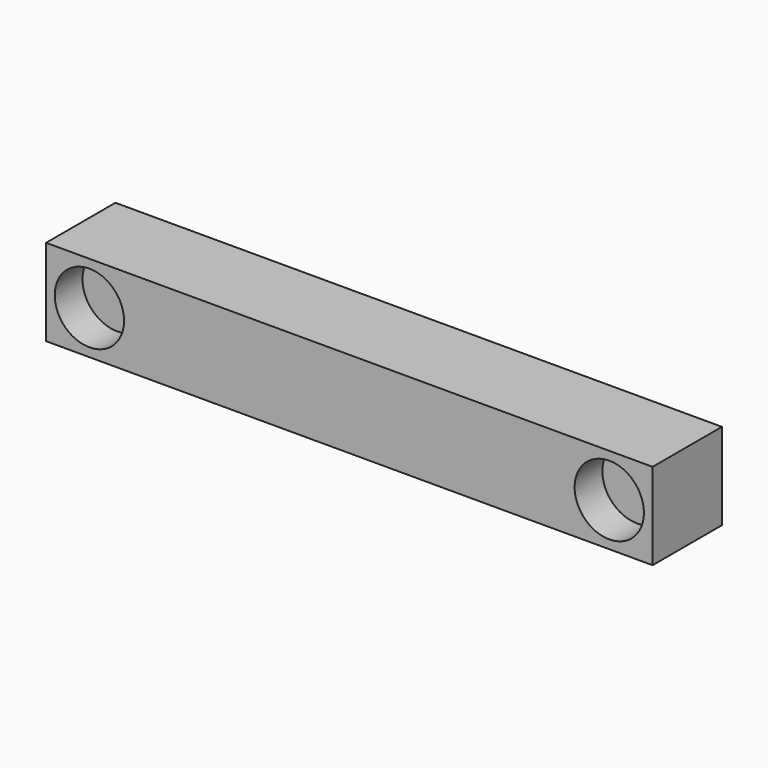
from build123d import *

# Parameters (mm, degrees)
F0_W     = 70
F0_H     = 10
F1_DEPTH = 10
F2_R     = 4
F3_DEPTH = 4


with BuildPart() as f1:
    # F0 (on Top) → F1 (new body)
    with BuildSketch(Plane.XY):
        with Locations((0, 7.5)):
            Rectangle(F0_W, F0_H)
    extrude(amount=F1_DEPTH)

    # F2 (on face) → F3 (cut)
    with BuildSketch(Plane.XZ.offset(-2.5)):
        with Locations((30, 5)):
            Circle(F2_R)
        with Locations((-30, 5)):
            Circle(F2_R)
    extrude(amount=-F3_DEPTH, mode=Mode.SUBTRACT)


solid = f1.part
